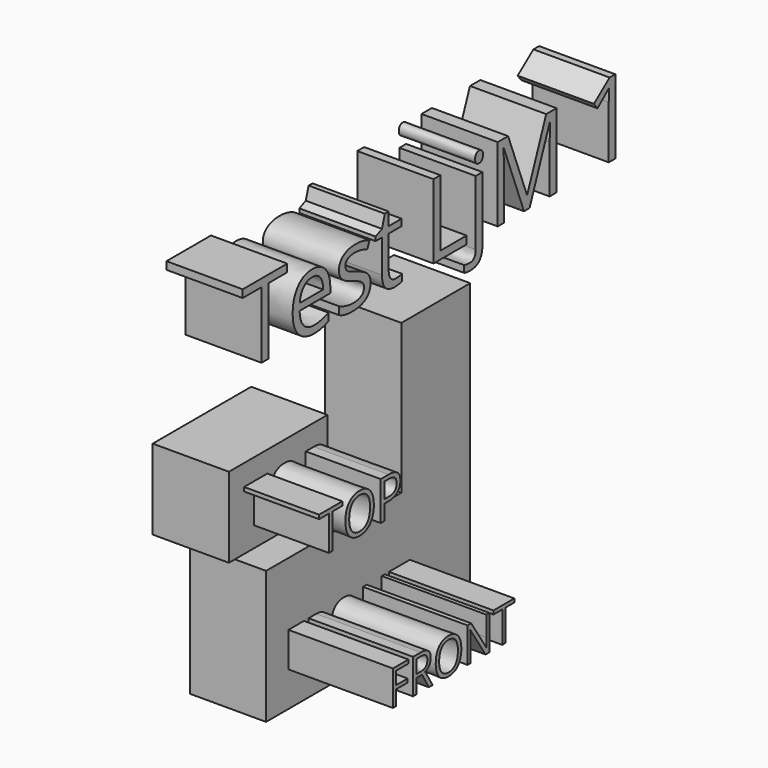
from build123d import *

# Parameters (mm, degrees)
F0_W         = 15.1579957455
F0_H         = 44.3110018969
F0_W_2       = 56.3495904207
F0_W_3       = 41.0301871598
F0_H_2       = 26.6962274909
F0_TEXT_SIZE = 34.648573233
F1_DEPTH     = 25.4
F2_TEXT_SIZE = 16.2429564322
F3_DEPTH     = 34.8262861371
F4_TEXT_SIZE = 18.0530193676
F5_DEPTH     = 25


# Not quite as in the source:
# - Text() gives the source's letters only with a copy of the font that has no kerning and outlines rounded to 1/6400 em; it was checked with that copy


with BuildPart() as f1:
    # F0 (on Right) → F1 (new body)
    with BuildSketch(Plane.YZ):
        Polygon((45.9561087191, 0), (45.9561087191, -44.3110018969), (30.7981129736, -44.3110018969), (30.7981129736, -55.0806969404), (59.4780147076, -55.0806969404), (59.4780147076, 49.8297810555), (30.7981129736, 49.8297810555), (30.7981129736, 0), align=None)
        with Locations((38.3771108463, -22.1555009484)):
            Rectangle(F0_W, F0_H)
        with Locations((2.6233177632, -22.1555009484)):
            Rectangle(F0_W_2, F0_H)
        with Locations((-20.5150935799, 22.0139883459)):
            Rectangle(F0_W_3, F0_H_2)
        with Locations((-35.5938784778, 61.8114322424)):
            Text('Test LjM 1', F0_TEXT_SIZE, font='Open Sans', text_align=(TextAlign.LEFT, TextAlign.BOTTOM))
    extrude(amount=F1_DEPTH)

    # F2 (on face) → F3 (join)
    with BuildSketch(Plane.YZ.offset(25.4)):
        with Locations((-17.8402662277, -32.6838679612)):
            Text('FRONT', F2_TEXT_SIZE, font='Open Sans', text_align=(TextAlign.LEFT, TextAlign.BOTTOM))
    extrude(amount=F3_DEPTH)

    # F4 (on face) → F5 (join)
    with BuildSketch(Plane.YZ.offset(25.4)):
        with Locations((-34.8592437804, 15.4425287619)):
            Text('TOP', F4_TEXT_SIZE, font='Open Sans', text_align=(TextAlign.LEFT, TextAlign.BOTTOM))
    extrude(amount=F5_DEPTH)


solid = f1.part
